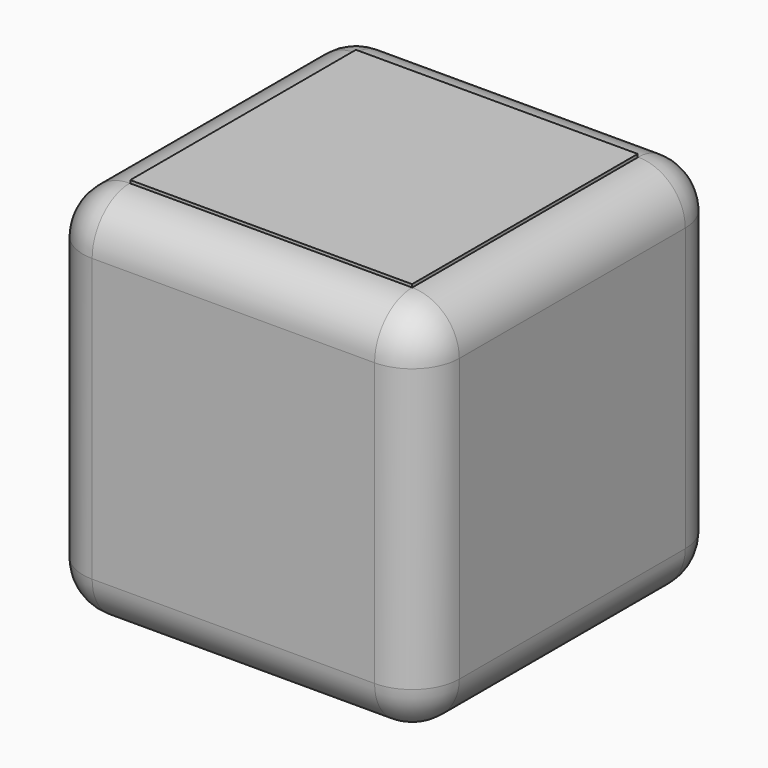
from build123d import *

# Parameters (mm, degrees)
F0_W     = 50.8120395243
F0_H     = 50.8120395243
F1_DEPTH = 50.8
F2_R     = 6.35
F3_T     = -5.08
F5_START = 49.53
F4_W     = 38.0277968943
F4_H     = 38.0652435124
F5_DEPTH = 1.651


# Not quite as in the source:
# - a shell that OpenCascade refuses in one call is made with other operations: the cavity is built on its own and cut out


with BuildPart() as f1:
    # F0 (on Top) → F1 (new body)
    with BuildSketch(Plane.XY):
        Rectangle(F0_W, F0_H)
    extrude(amount=F1_DEPTH)

    # F2
    f2_edges = [f1.edges().sort_by_distance(p)[0] for p in [
        (0, -25.40602, 50.8),
        (25.40602, 0, 50.8),
        (25.40602, -25.40602, 25.4),
        (25.40602, 25.40602, 25.4),
        (25.40602, 0, 0),
        (0, -25.40602, 0),
        (-25.40602, 0, 50.8),
        (0, 25.40602, 50.8),
        (-25.40602, -25.40602, 25.4),
        (-25.40602, 25.40602, 25.4),
        (0, 25.40602, 0),
        (-25.40602, 0, 0),
    ]]
    fillet(f2_edges, radius=F2_R)

    # F3: a shell. OpenCascade refuses it in one call, so the cavity is built on its own and cut out:
    # the body offset inwards by the wall thickness, plus a prism from it out through each open face.
    f3_core = offset(f1.part, amount=F3_T, mode=Mode.PRIVATE)
    f3_exits = [f3_core.faces().sort_by_distance(p)[0] for p in [
        (0, 0, 45.72),
    ]]
    add(f3_core, mode=Mode.SUBTRACT)
    extrude(f3_exits, amount=-F3_T, mode=Mode.SUBTRACT)


with BuildPart() as f5:
    # F4 (on Top) → F5 (new body)
    with BuildSketch(Plane.XY.offset(F5_START)):
        Rectangle(F4_W, F4_H)
    extrude(amount=F5_DEPTH)


solid = Compound([f1.part, f5.part])
